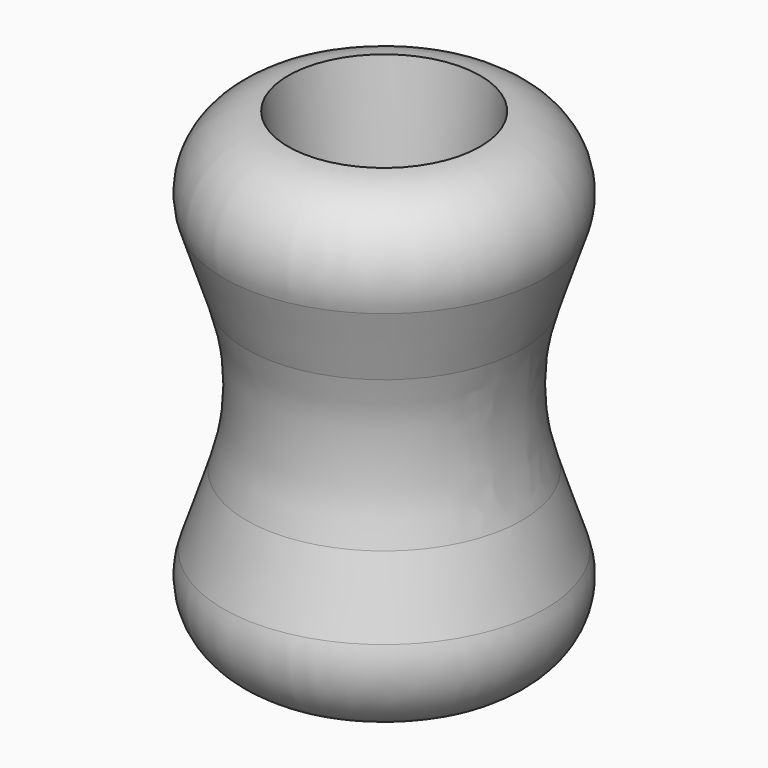
from build123d import *

# Parameters (mm, degrees)
F3_R = 5


# Not quite as in the source:
# - a fillet or chamfer that OpenCascade refuses, or shapes differently, is made with other operations: its cross-section is extruded or revolved along the edge and cut away or added


with BuildPart() as f1:
    # F0 (on Front) → F1 (revolve)
    with BuildSketch(Plane.XZ):
        Polygon((4, 11.2420413941), (2, 11.2420413941), (1.5147400554, 6.2420413941), (2, 1.2420413941), (4, 1.2420413941), (2.3485091515, 6.2420413941), align=None)
    revolve(axis=Axis((0, 0, 6.2420413941), (0, 0, 1)))

    # F2: fillet of radius 1.5 on 2 edges, made by hand

    # F2_s1 → F2_t2 (revolve, cut)
    with BuildSketch(Plane.XZ):
        with BuildLine():
            ThreePointArc((3.3497763701, 9.2734454721), (3.162587688, 10.592136722), (2, 11.2420413941))
            Line((2, 11.2420413941), (4, 11.2420413941))
            Line((4, 11.2420413941), (3.3497763701, 9.2734454721))
        make_face()
    revolve(axis=Axis((0, 0, 11.2420413941), (0, 0, 1)), mode=Mode.SUBTRACT)

    # F2_s3 → F2_t4 (revolve, cut)
    with BuildSketch(Plane.XZ):
        with BuildLine():
            ThreePointArc((2, 1.2420413941), (3.162587688, 1.8919460662), (3.3497763701, 3.2106373161))
            Line((3.3497763701, 3.2106373161), (4, 1.2420413941))
            Line((4, 1.2420413941), (2, 1.2420413941))
        make_face()
    revolve(axis=Axis((0, 0, 1.2420413941), (0, 0, 1)), mode=Mode.SUBTRACT)

    # F3
    f3_edges = [f1.edges().sort_by_distance(p)[0] for p in [
        (-2.348509, 0, 6.242041),
    ]]
    fillet(f3_edges, radius=F3_R)


solid = f1.part
